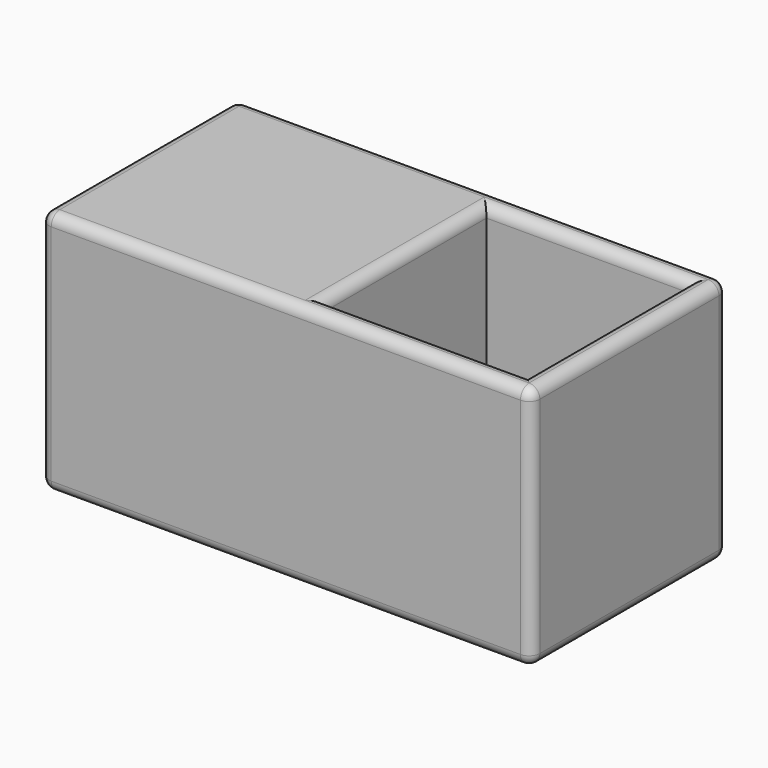
from build123d import *

# Parameters (mm, degrees)
F1_DEPTH              = 34.2
F2_W                  = 28.2
F2_H                  = 28.2
F3_DEPTH              = 31.2
F4_W                  = 34.2
F4_H                  = 34.2
F5_DEPTH              = 34.2
F6_W                  = 28.2
F6_H                  = 28.2
F7_DEPTH              = 31.2
F10_D                 = 3.3
F10_DEPTH             = 25
F10_CSINK_D           = 6.72
F10_CSINK_ANGLE       = 90
F10_TIP               = 0.9914200214
F10_ON_F9_D           = 3.3
F10_ON_F9_DEPTH       = 25
F10_ON_F9_CSINK_D     = 6.72
F10_ON_F9_CSINK_ANGLE = 90
F10_ON_F9_TIP         = 0.9914200214
F11_R                 = 1.49999
F12_W                 = 5
F12_H                 = 5
F13_DEPTH             = 2.5


# Not quite as in the source:
# - a fillet or chamfer is up to 0.001 mm smaller than in the source, because OpenCascade refuses the exact size
# - a feature names something its author has since deleted; it is built from what else it names


with BuildPart() as f1:
    # F0 (on Top) → F1 (new body)
    with BuildSketch(Plane.XY):
        Polygon((-34.2, 0), (-8, 0), (0, 0), (0, 34.2), (-34.2, 34.2), align=None)
    extrude(amount=F1_DEPTH)

    # F2 (on face) → F3 (cut)
    with BuildSketch(Plane.XY.offset(34.2)):
        with Locations((-17.1, 17.1)):
            Rectangle(F2_W, F2_H)
    extrude(amount=-F3_DEPTH, mode=Mode.SUBTRACT)

    # F4 (on face) → F5 (join)
    with BuildSketch(Plane(origin=(-34.2, 0, 0), x_dir=(0, -1, 0), z_dir=(-1, 0, 0))):
        with Locations((-17.1, 17.1)):
            Rectangle(F4_W, F4_H)
    extrude(amount=F5_DEPTH)

    # F6 (on face) → F7 (cut)
    with BuildSketch(Plane(origin=(-68.4, 0, 0), x_dir=(0, -1, 0), z_dir=(-1, 0, 0))):
        with Locations((-17.1, 17.1)):
            Rectangle(F6_W, F6_H)
    extrude(amount=-F7_DEPTH, mode=Mode.SUBTRACT)

    # F10
    with Locations(Plane(origin=(0, 34.2, 0), x_dir=(-1, 0, 0), z_dir=(0, 1, 0))):
        with Locations((17.05, 17.1), (51.35, 17.1)):
            CounterSinkHole(F10_D / 2, F10_CSINK_D / 2, depth=F10_DEPTH, counter_sink_angle=F10_CSINK_ANGLE)
            with Locations((0, 0, -(F10_DEPTH + F10_TIP / 2))):  # 118° drill point
                Cone(0, F10_D / 2, F10_TIP, mode=Mode.SUBTRACT)

    # F10 on F9
    with Locations(Plane(origin=(-37.2, 0, 0), x_dir=(0, -1, 0), z_dir=(-1, 0, 0))):
        with Locations((-17.1, 17.1)):
            CounterSinkHole(F10_ON_F9_D / 2, F10_ON_F9_CSINK_D / 2, depth=F10_ON_F9_DEPTH, counter_sink_angle=F10_ON_F9_CSINK_ANGLE)
            with Locations((0, 0, -(F10_ON_F9_DEPTH + F10_ON_F9_TIP / 2))):  # 118° drill point
                Cone(0, F10_ON_F9_D / 2, F10_ON_F9_TIP, mode=Mode.SUBTRACT)

    # F11 (radius 1.5 in the source; OpenCascade refuses exactly that, so slightly less here)
    f11_edges = [f1.edges().sort_by_distance(p)[0] for p in [
        (-31.2, 17.1, 34.2),
        (-17.1, 31.2, 34.2),
        (-17.1, 31.2, 3),
        (0, 17.1, 34.2),
        (-34.2, 0, 34.2),
        (-68.4, 17.1, 34.2),
        (-34.2, 34.2, 34.2),
        (0, 34.2, 17.1),
        (-68.4, 17.1, 31.2),
        (-68.4, 0, 17.1),
        (-68.4, 3, 17.1),
        (-68.4, 31.2, 17.1),
        (-68.4, 34.2, 17.1),
        (-68.4, 17.1, 3),
        (-68.4, 17.1, 0),
        (-34.2, 0, 0),
        (-34.2, 34.2, 0),
        (0, 0, 17.1),
        (-3, 17.1, 34.2),
        (-17.1, 3, 34.2),
        (0, 17.1, 0),
    ]]
    fillet(f11_edges, radius=F11_R)

    # F12 (on face) → F13 (cut)
    with BuildSketch(Plane(origin=(0, 34.2, 0), x_dir=(-1, 0, 0), z_dir=(0, 1, 0))):
        with Locations((14.6, 6.5)):
            Rectangle(F12_W, F12_H)
    extrude(amount=-F13_DEPTH, mode=Mode.SUBTRACT)


solid = f1.part
